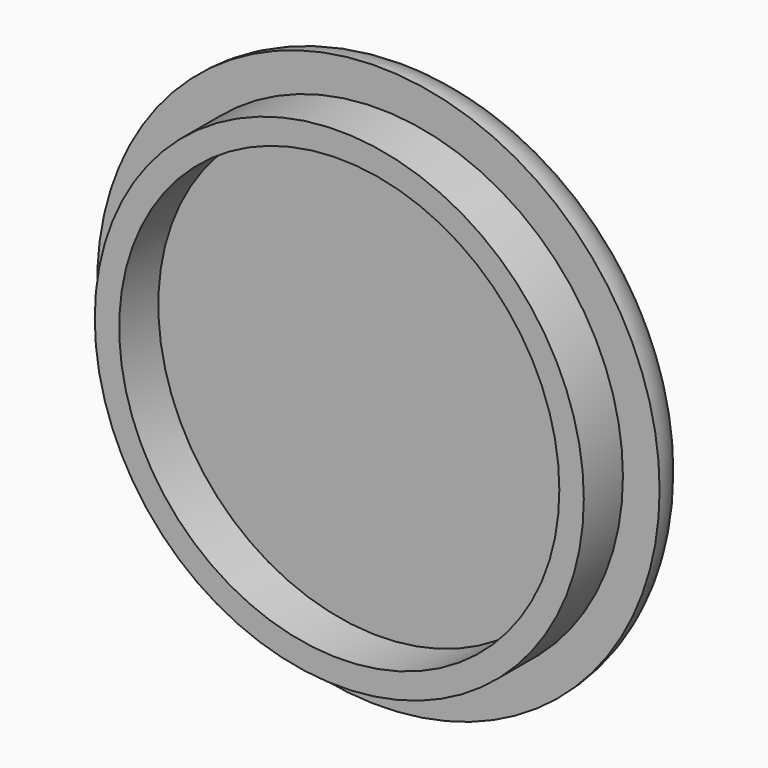
from build123d import *

# Parameters (mm, degrees)
F0_R     = 11.5
F1_DEPTH = 2
F2_R     = 10
F2_R_2   = 9
F3_DEPTH = 2
F4_R     = 1.99999


# Not quite as in the source:
# - a fillet or chamfer is up to 0.001 mm smaller than in the source, because OpenCascade refuses the exact size


with BuildPart() as f1:
    # F0 (on Front) → F1 (new body)
    with BuildSketch(Plane.XZ):
        Circle(F0_R)
    extrude(amount=F1_DEPTH)

    # F2 (on face) → F3 (join)
    with BuildSketch(Plane.XZ.offset(2)):
        Circle(F2_R)
        Circle(F2_R_2, mode=Mode.SUBTRACT)
    extrude(amount=F3_DEPTH)

    # F4 (radius 2 in the source; OpenCascade refuses exactly that, so slightly less here)
    f4_edges = [f1.edges().sort_by_distance(p)[0] for p in [
        (-11.5, 0, 0),
    ]]
    fillet(f4_edges, radius=F4_R)


solid = f1.part
